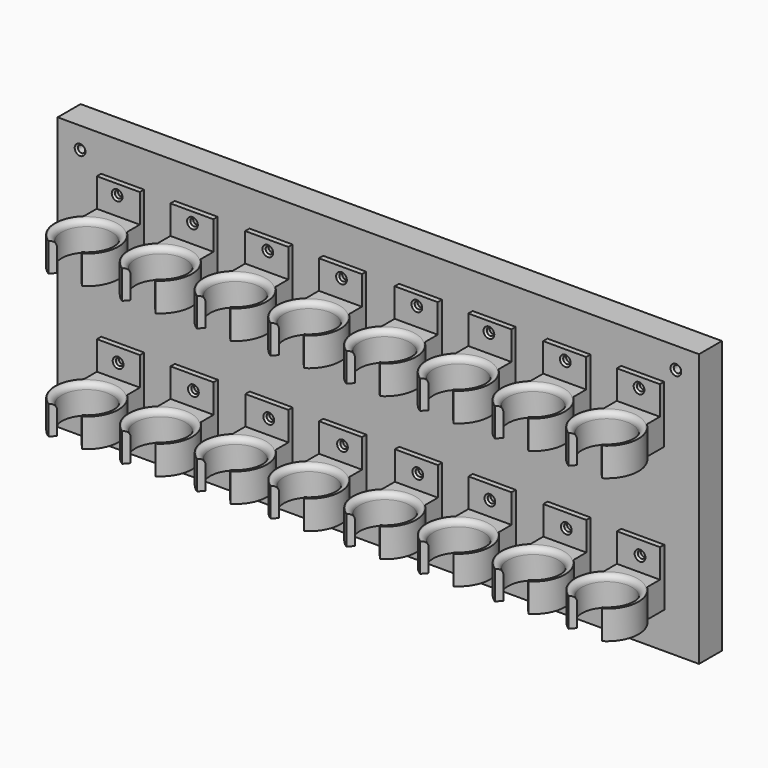
from build123d import *

# Parameters (mm, degrees)
F1_DEPTH          = 25.4
F4_DEPTH          = 25.4
F0_W              = 38.1424913003
F0_H              = 4.7625
F5_DEPTH          = 50.8
F3_W              = 38.1424913003
F3_H              = 4.7625
F6_DEPTH          = 50.8
F9_D              = 6.35
F9_CSINK_D        = 9.525
F9_CSINK_ANGLE    = 90
F9_2_D            = 6.35
F9_2_CSINK_D      = 9.525
F9_2_CSINK_ANGLE  = 90
F9_3_D            = 6.35
F9_3_CSINK_D      = 9.525
F9_3_CSINK_ANGLE  = 90
F9_4_D            = 6.35
F9_4_CSINK_D      = 9.525
F9_4_CSINK_ANGLE  = 90
F9_5_D            = 6.35
F9_5_CSINK_D      = 9.525
F9_5_CSINK_ANGLE  = 90
F9_6_D            = 6.35
F9_6_CSINK_D      = 9.525
F9_6_CSINK_ANGLE  = 90
F9_7_D            = 6.35
F9_7_CSINK_D      = 9.525
F9_7_CSINK_ANGLE  = 90
F9_8_D            = 6.35
F9_8_CSINK_D      = 9.525
F9_8_CSINK_ANGLE  = 90
F12_D             = 6.35
F12_CSINK_D       = 9.525
F12_CSINK_ANGLE   = 90
F12_2_D           = 6.35
F12_2_CSINK_D     = 9.525
F12_2_CSINK_ANGLE = 90
F12_3_D           = 6.35
F12_3_CSINK_D     = 9.525
F12_3_CSINK_ANGLE = 90
F12_4_D           = 6.35
F12_4_CSINK_D     = 9.525
F12_4_CSINK_ANGLE = 90
F12_5_D           = 6.35
F12_5_CSINK_D     = 9.525
F12_5_CSINK_ANGLE = 90
F12_6_D           = 6.35
F12_6_CSINK_D     = 9.525
F12_6_CSINK_ANGLE = 90
F12_7_D           = 6.35
F12_7_CSINK_D     = 9.525
F12_7_CSINK_ANGLE = 90
F12_8_D           = 6.35
F12_8_CSINK_D     = 9.525
F12_8_CSINK_ANGLE = 90
F13_R             = 5.08
F13_2_R           = 5.08
F13_3_R           = 5.08
F13_4_R           = 5.08
F13_5_R           = 5.08
F13_6_R           = 5.08
F13_7_R           = 5.08
F13_8_R           = 5.08
F13_9_R           = 5.08
F13_10_R          = 5.08
F13_11_R          = 5.08
F13_12_R          = 5.08
F13_13_R          = 5.08
F13_14_R          = 5.08
F13_15_R          = 5.08
F13_16_R          = 5.08
F15_W             = 568.5065984726
F15_H             = 241.7119890451
F16_DEPTH         = 25.4
F18_D             = 6.35
F18_CSINK_D       = 9.525
F18_CSINK_ANGLE   = 90


# Not quite as in the source:
# - a feature names something its author has since deleted; it is built from what else it names


with BuildPart() as f1:
    # F0 (on Top) → F1 (new body)
    with BuildSketch(Plane.XY):
        with BuildLine():
            Line((-236.2981056251, -12.180712776), (-274.4405969254, -12.180712776))
            Line((-274.4405969254, -12.180712776), (-274.4405969254, -16.943212776))
            Line((-274.4405969254, -16.943212776), (-274.4405969254, -26.468212776))
            ThreePointArc((-274.4405969254, -26.468212776), (-255.3693512752, -19.0188201484), (-236.2981056251, -26.468212776))
            Line((-236.2981056251, -26.468212776), (-236.2981056251, -16.943212776))
            Line((-236.2981056251, -16.943212776), (-236.2981056251, -12.180712776))
        make_face()
        with BuildLine():
            ThreePointArc((-236.2981056251, -26.468212776), (-255.3693512752, -19.0188201484), (-274.4405969254, -26.468212776))
            ThreePointArc((-274.4405969254, -26.468212776), (-283.3824945845, -49.791985495), (-270.2462375164, -71.0380359006))
            Line((-270.2462375164, -71.0380359006), (-266.2968452207, -66.5087844903))
            ThreePointArc((-266.2968452207, -66.5087844903), (-255.3693512752, -24.9307356072), (-244.4418573298, -66.5087844903))
            Line((-244.4418573298, -66.5087844903), (-240.4924650341, -71.0380359006))
            ThreePointArc((-240.4924650341, -71.0380359006), (-227.356207966, -49.791985495), (-236.2981056251, -26.468212776))
        make_face()
    extrude(amount=F1_DEPTH)

    # F0 (on Top) → F5 (join)
    with BuildSketch(Plane.XY):
        with Locations((-255.3693512752, -9.799462776)):
            Rectangle(F0_W, F0_H)
    extrude(amount=F5_DEPTH)

    # F9 (through all)
    with Locations(Plane.XZ.offset(12.180712776)):
        with Locations((-57.5012685731, 41.7619496584), (-256.4041018486, 41.7619496584), (-122.8343173862, 41.7619496584), (-189.6192133427, 41.7619496584), (206.250667572, 41.7619496584), (73.1648281217, 41.7619496584), (9.2836245894, 41.7619496584), (140.9176290035, 41.7619496584)):
            CounterSinkHole(F9_D / 2, F9_CSINK_D / 2, counter_sink_angle=F9_CSINK_ANGLE)

    # F13
    f13_edges = [f1.edges().sort_by_distance(p)[0] for p in [
        (-255.369351, -24.930736, 25.4),
    ]]
    fillet(f13_edges, radius=F13_R)



with BuildPart() as f1b:
    # F0 (on Top) → F1, piece 2 (new body)
    with BuildSketch(Plane.XY):
        with BuildLine():
            ThreePointArc((-171.0200906615, -26.468212776), (-190.0913363116, -19.0188201484), (-209.1625819618, -26.468212776))
            ThreePointArc((-209.1625819618, -26.468212776), (-218.1044796209, -49.791985495), (-204.9682225528, -71.0380359006))
            Line((-204.9682225528, -71.0380359006), (-201.0188302571, -66.5087844903))
            ThreePointArc((-201.0188302571, -66.5087844903), (-190.0913363116, -24.9307356072), (-179.1638423661, -66.5087844903))
            Line((-179.1638423661, -66.5087844903), (-175.2144500705, -71.0380359006))
            ThreePointArc((-175.2144500705, -71.0380359006), (-162.0781930024, -49.791985495), (-171.0200906615, -26.468212776))
        make_face()
        with BuildLine():
            Line((-171.0200906615, -12.180712776), (-209.1625819618, -12.180712776))
            Line((-209.1625819618, -12.180712776), (-209.1625819618, -16.943212776))
            Line((-209.1625819618, -16.943212776), (-209.1625819618, -26.468212776))
            ThreePointArc((-209.1625819618, -26.468212776), (-190.0913363116, -19.0188201484), (-171.0200906615, -26.468212776))
            Line((-171.0200906615, -26.468212776), (-171.0200906615, -16.943212776))
            Line((-171.0200906615, -16.943212776), (-171.0200906615, -12.180712776))
        make_face()
    extrude(amount=F1_DEPTH)

    # F0 (on Top) → F5, piece 2 (join)
    with BuildSketch(Plane.XY):
        with Locations((-190.0913363116, -9.799462776)):
            Rectangle(F0_W, F0_H)
    extrude(amount=F5_DEPTH)

    # F9#2 (through all)
    with Locations(Plane.XZ.offset(12.180712776)):
        with Locations((-57.5012685731, 41.7619496584), (-256.4041018486, 41.7619496584), (-122.8343173862, 41.7619496584), (-189.6192133427, 41.7619496584), (206.250667572, 41.7619496584), (73.1648281217, 41.7619496584), (9.2836245894, 41.7619496584), (140.9176290035, 41.7619496584)):
            CounterSinkHole(F9_2_D / 2, F9_2_CSINK_D / 2, counter_sink_angle=F9_2_CSINK_ANGLE)

    # F13#2
    f13_2_edges = [f1b.edges().sort_by_distance(p)[0] for p in [
        (-190.091336, -24.930736, 25.4),
    ]]
    fillet(f13_2_edges, radius=F13_2_R)


with BuildPart() as f1c:
    # F0 (on Top) → F1, piece 3 (new body)
    with BuildSketch(Plane.XY):
        with BuildLine():
            Line((-104.6902751007, -12.180712776), (-142.8327664009, -12.180712776))
            Line((-142.8327664009, -12.180712776), (-142.8327664009, -16.943212776))
            Line((-142.8327664009, -16.943212776), (-142.8327664009, -26.468212776))
            ThreePointArc((-142.8327664009, -26.468212776), (-123.7615207508, -19.0188201484), (-104.6902751007, -26.468212776))
            Line((-104.6902751007, -26.468212776), (-104.6902751007, -16.943212776))
            Line((-104.6902751007, -16.943212776), (-104.6902751007, -12.180712776))
        make_face()
        with BuildLine():
            ThreePointArc((-104.6902751007, -26.468212776), (-123.7615207508, -19.0188201484), (-142.8327664009, -26.468212776))
            ThreePointArc((-142.8327664009, -26.468212776), (-151.7746640601, -49.791985495), (-138.638406992, -71.0380359006))
            Line((-138.638406992, -71.0380359006), (-134.6890146963, -66.5087844903))
            ThreePointArc((-134.6890146963, -66.5087844903), (-123.7615207508, -24.9307356072), (-112.8340268053, -66.5087844903))
            Line((-112.8340268053, -66.5087844903), (-108.8846345096, -71.0380359006))
            ThreePointArc((-108.8846345096, -71.0380359006), (-95.7483774415, -49.791985495), (-104.6902751007, -26.468212776))
        make_face()
    extrude(amount=F1_DEPTH)

    # F0 (on Top) → F5, piece 3 (join)
    with BuildSketch(Plane.XY):
        with Locations((-123.7615207508, -9.799462776)):
            Rectangle(F0_W, F0_H)
    extrude(amount=F5_DEPTH)

    # F9#3 (through all)
    with Locations(Plane.XZ.offset(12.180712776)):
        with Locations((-57.5012685731, 41.7619496584), (-256.4041018486, 41.7619496584), (-122.8343173862, 41.7619496584), (-189.6192133427, 41.7619496584), (206.250667572, 41.7619496584), (73.1648281217, 41.7619496584), (9.2836245894, 41.7619496584), (140.9176290035, 41.7619496584)):
            CounterSinkHole(F9_3_D / 2, F9_3_CSINK_D / 2, counter_sink_angle=F9_3_CSINK_ANGLE)

    # F13#3
    f13_3_edges = [f1c.edges().sort_by_distance(p)[0] for p in [
        (-123.761521, -24.930736, 25.4),
    ]]
    fillet(f13_3_edges, radius=F13_3_R)


with BuildPart() as f1d:
    # F0 (on Top) → F1, piece 4 (new body)
    with BuildSketch(Plane.XY):
        with BuildLine():
            ThreePointArc((-39.412260137, -26.468212776), (-58.4835057872, -19.0188201484), (-77.5547514373, -26.468212776))
            ThreePointArc((-77.5547514373, -26.468212776), (-86.4966490964, -49.791985495), (-73.3603920283, -71.0380359006))
            Line((-73.3603920283, -71.0380359006), (-69.4109997327, -66.5087844903))
            ThreePointArc((-69.4109997327, -66.5087844903), (-58.4835057872, -24.9307356072), (-47.5560118417, -66.5087844903))
            Line((-47.5560118417, -66.5087844903), (-43.606619546, -71.0380359006))
            ThreePointArc((-43.606619546, -71.0380359006), (-30.4703624779, -49.791985495), (-39.412260137, -26.468212776))
        make_face()
        with BuildLine():
            Line((-39.412260137, -12.180712776), (-77.5547514373, -12.180712776))
            Line((-77.5547514373, -12.180712776), (-77.5547514373, -16.943212776))
            Line((-77.5547514373, -16.943212776), (-77.5547514373, -26.468212776))
            ThreePointArc((-77.5547514373, -26.468212776), (-58.4835057872, -19.0188201484), (-39.412260137, -26.468212776))
            Line((-39.412260137, -26.468212776), (-39.412260137, -16.943212776))
            Line((-39.412260137, -16.943212776), (-39.412260137, -12.180712776))
        make_face()
    extrude(amount=F1_DEPTH)

    # F0 (on Top) → F5, piece 4 (join)
    with BuildSketch(Plane.XY):
        with Locations((-58.4835057872, -9.799462776)):
            Rectangle(F0_W, F0_H)
    extrude(amount=F5_DEPTH)

    # F9#4 (through all)
    with Locations(Plane.XZ.offset(12.180712776)):
        with Locations((-57.5012685731, 41.7619496584), (-256.4041018486, 41.7619496584), (-122.8343173862, 41.7619496584), (-189.6192133427, 41.7619496584), (206.250667572, 41.7619496584), (73.1648281217, 41.7619496584), (9.2836245894, 41.7619496584), (140.9176290035, 41.7619496584)):
            CounterSinkHole(F9_4_D / 2, F9_4_CSINK_D / 2, counter_sink_angle=F9_4_CSINK_ANGLE)

    # F13#4
    f13_4_edges = [f1d.edges().sort_by_distance(p)[0] for p in [
        (-58.483506, -24.930736, 25.4),
    ]]
    fillet(f13_4_edges, radius=F13_4_R)


with BuildPart() as f1e:
    # F0 (on Top) → F1, piece 5 (new body)
    with BuildSketch(Plane.XY):
        with BuildLine():
            ThreePointArc((27.8059840746, -26.468212776), (8.7347384244, -19.0188201484), (-10.3365072257, -26.468212776))
            ThreePointArc((-10.3365072257, -26.468212776), (-19.2784048848, -49.791985495), (-6.1421478167, -71.0380359006))
            Line((-6.1421478167, -71.0380359006), (-2.192755521, -66.5087844903))
            ThreePointArc((-2.192755521, -66.5087844903), (8.7347384244, -24.9307356072), (19.6622323699, -66.5087844903))
            Line((19.6622323699, -66.5087844903), (23.6116246656, -71.0380359006))
            ThreePointArc((23.6116246656, -71.0380359006), (36.7478817337, -49.791985495), (27.8059840746, -26.468212776))
        make_face()
        with BuildLine():
            Line((27.8059840746, -12.180712776), (-10.3365072257, -12.180712776))
            Line((-10.3365072257, -12.180712776), (-10.3365072257, -16.943212776))
            Line((-10.3365072257, -16.943212776), (-10.3365072257, -26.468212776))
            ThreePointArc((-10.3365072257, -26.468212776), (8.7347384244, -19.0188201484), (27.8059840746, -26.468212776))
            Line((27.8059840746, -26.468212776), (27.8059840746, -16.943212776))
            Line((27.8059840746, -16.943212776), (27.8059840746, -12.180712776))
        make_face()
    extrude(amount=F1_DEPTH)

    # F0 (on Top) → F5, piece 5 (join)
    with BuildSketch(Plane.XY):
        with Locations((8.7347384244, -9.799462776)):
            Rectangle(F0_W, F0_H)
    extrude(amount=F5_DEPTH)

    # F9#5 (through all)
    with Locations(Plane.XZ.offset(12.180712776)):
        with Locations((-57.5012685731, 41.7619496584), (-256.4041018486, 41.7619496584), (-122.8343173862, 41.7619496584), (-189.6192133427, 41.7619496584), (206.250667572, 41.7619496584), (73.1648281217, 41.7619496584), (9.2836245894, 41.7619496584), (140.9176290035, 41.7619496584)):
            CounterSinkHole(F9_5_D / 2, F9_5_CSINK_D / 2, counter_sink_angle=F9_5_CSINK_ANGLE)

    # F13#5
    f13_5_edges = [f1e.edges().sort_by_distance(p)[0] for p in [
        (8.734738, -24.930736, 25.4),
    ]]
    fillet(f13_5_edges, radius=F13_5_R)


with BuildPart() as f1f:
    # F0 (on Top) → F1, piece 6 (new body)
    with BuildSketch(Plane.XY):
        with BuildLine():
            ThreePointArc((93.0839990382, -26.468212776), (74.0127533881, -19.0188201484), (54.9415077379, -26.468212776))
            ThreePointArc((54.9415077379, -26.468212776), (45.9996100788, -49.791985495), (59.1358671469, -71.0380359006))
            Line((59.1358671469, -71.0380359006), (63.0852594426, -66.5087844903))
            ThreePointArc((63.0852594426, -66.5087844903), (74.0127533881, -24.9307356072), (84.9402473335, -66.5087844903))
            Line((84.9402473335, -66.5087844903), (88.8896396292, -71.0380359006))
            ThreePointArc((88.8896396292, -71.0380359006), (102.0258966973, -49.791985495), (93.0839990382, -26.468212776))
        make_face()
        with BuildLine():
            Line((93.0839990382, -12.180712776), (54.9415077379, -12.180712776))
            Line((54.9415077379, -12.180712776), (54.9415077379, -16.943212776))
            Line((54.9415077379, -16.943212776), (54.9415077379, -26.468212776))
            ThreePointArc((54.9415077379, -26.468212776), (74.0127533881, -19.0188201484), (93.0839990382, -26.468212776))
            Line((93.0839990382, -26.468212776), (93.0839990382, -16.943212776))
            Line((93.0839990382, -16.943212776), (93.0839990382, -12.180712776))
        make_face()
    extrude(amount=F1_DEPTH)

    # F0 (on Top) → F5, piece 6 (join)
    with BuildSketch(Plane.XY):
        with Locations((74.0127533881, -9.799462776)):
            Rectangle(F0_W, F0_H)
    extrude(amount=F5_DEPTH)

    # F9#6 (through all)
    with Locations(Plane.XZ.offset(12.180712776)):
        with Locations((-57.5012685731, 41.7619496584), (-256.4041018486, 41.7619496584), (-122.8343173862, 41.7619496584), (-189.6192133427, 41.7619496584), (206.250667572, 41.7619496584), (73.1648281217, 41.7619496584), (9.2836245894, 41.7619496584), (140.9176290035, 41.7619496584)):
            CounterSinkHole(F9_6_D / 2, F9_6_CSINK_D / 2, counter_sink_angle=F9_6_CSINK_ANGLE)

    # F13#6
    f13_6_edges = [f1f.edges().sort_by_distance(p)[0] for p in [
        (74.012753, -24.930736, 25.4),
    ]]
    fillet(f13_6_edges, radius=F13_6_R)


with BuildPart() as f1g:
    # F0 (on Top) → F1, piece 7 (new body)
    with BuildSketch(Plane.XY):
        with BuildLine():
            ThreePointArc((159.413814599, -26.468212776), (140.3425689489, -19.0188201484), (121.2713232988, -26.468212776))
            ThreePointArc((121.2713232988, -26.468212776), (112.3294256396, -49.791985495), (125.4656827077, -71.0380359006))
            Line((125.4656827077, -71.0380359006), (129.4150750034, -66.5087844903))
            ThreePointArc((129.4150750034, -66.5087844903), (140.3425689489, -24.9307356072), (151.2700628944, -66.5087844903))
            Line((151.2700628944, -66.5087844903), (155.2194551901, -71.0380359006))
            ThreePointArc((155.2194551901, -71.0380359006), (168.3557122582, -49.791985495), (159.413814599, -26.468212776))
        make_face()
        with BuildLine():
            Line((159.413814599, -12.180712776), (121.2713232988, -12.180712776))
            Line((121.2713232988, -12.180712776), (121.2713232988, -16.943212776))
            Line((121.2713232988, -16.943212776), (121.2713232988, -26.468212776))
            ThreePointArc((121.2713232988, -26.468212776), (140.3425689489, -19.0188201484), (159.413814599, -26.468212776))
            Line((159.413814599, -26.468212776), (159.413814599, -16.943212776))
            Line((159.413814599, -16.943212776), (159.413814599, -12.180712776))
        make_face()
    extrude(amount=F1_DEPTH)

    # F0 (on Top) → F5, piece 7 (join)
    with BuildSketch(Plane.XY):
        with Locations((140.3425689489, -9.799462776)):
            Rectangle(F0_W, F0_H)
    extrude(amount=F5_DEPTH)

    # F9#7 (through all)
    with Locations(Plane.XZ.offset(12.180712776)):
        with Locations((-57.5012685731, 41.7619496584), (-256.4041018486, 41.7619496584), (-122.8343173862, 41.7619496584), (-189.6192133427, 41.7619496584), (206.250667572, 41.7619496584), (73.1648281217, 41.7619496584), (9.2836245894, 41.7619496584), (140.9176290035, 41.7619496584)):
            CounterSinkHole(F9_7_D / 2, F9_7_CSINK_D / 2, counter_sink_angle=F9_7_CSINK_ANGLE)

    # F13#7
    f13_7_edges = [f1g.edges().sort_by_distance(p)[0] for p in [
        (140.342569, -24.930736, 25.4),
    ]]
    fillet(f13_7_edges, radius=F13_7_R)


with BuildPart() as f1h:
    # F0 (on Top) → F1, piece 8 (new body)
    with BuildSketch(Plane.XY):
        with BuildLine():
            ThreePointArc((224.6918295626, -26.468212776), (205.6205839125, -19.0188201484), (186.5493382624, -26.468212776))
            ThreePointArc((186.5493382624, -26.468212776), (177.6074406032, -49.791985495), (190.7436976713, -71.0380359006))
            Line((190.7436976713, -71.0380359006), (194.693089967, -66.5087844903))
            ThreePointArc((194.693089967, -66.5087844903), (205.6205839125, -24.9307356072), (216.548077858, -66.5087844903))
            Line((216.548077858, -66.5087844903), (220.4974701537, -71.0380359006))
            ThreePointArc((220.4974701537, -71.0380359006), (233.6337272218, -49.791985495), (224.6918295626, -26.468212776))
        make_face()
        with BuildLine():
            Line((224.6918295626, -12.180712776), (186.5493382624, -12.180712776))
            Line((186.5493382624, -12.180712776), (186.5493382624, -16.943212776))
            Line((186.5493382624, -16.943212776), (186.5493382624, -26.468212776))
            ThreePointArc((186.5493382624, -26.468212776), (205.6205839125, -19.0188201484), (224.6918295626, -26.468212776))
            Line((224.6918295626, -26.468212776), (224.6918295626, -16.943212776))
            Line((224.6918295626, -16.943212776), (224.6918295626, -12.180712776))
        make_face()
    extrude(amount=F1_DEPTH)

    # F0 (on Top) → F5, piece 8 (join)
    with BuildSketch(Plane.XY):
        with Locations((205.6205839125, -9.799462776)):
            Rectangle(F0_W, F0_H)
    extrude(amount=F5_DEPTH)

    # F9#8 (through all)
    with Locations(Plane.XZ.offset(12.180712776)):
        with Locations((-57.5012685731, 41.7619496584), (-256.4041018486, 41.7619496584), (-122.8343173862, 41.7619496584), (-189.6192133427, 41.7619496584), (206.250667572, 41.7619496584), (73.1648281217, 41.7619496584), (9.2836245894, 41.7619496584), (140.9176290035, 41.7619496584)):
            CounterSinkHole(F9_8_D / 2, F9_8_CSINK_D / 2, counter_sink_angle=F9_8_CSINK_ANGLE)

    # F13#8
    f13_8_edges = [f1h.edges().sort_by_distance(p)[0] for p in [
        (205.620584, -24.930736, 25.4),
    ]]
    fillet(f13_8_edges, radius=F13_8_R)


with BuildPart() as f4:
    # F3 (on offset) → F4 (new body)
    with BuildSketch(Plane.XY.offset(-127)):
        with BuildLine():
            Line((224.9779318576, -12.3800472473), (186.8354405573, -12.3800472473))
            Line((186.8354405573, -12.3800472473), (186.8354405573, -17.1425472473))
            Line((186.8354405573, -17.1425472473), (186.8354405573, -26.6675472473))
            ThreePointArc((186.8354405573, -26.6675472473), (205.9066862074, -19.2181546196), (224.9779318576, -26.6675472473))
            Line((224.9779318576, -26.6675472473), (224.9779318576, -17.1425472473))
            Line((224.9779318576, -17.1425472473), (224.9779318576, -12.3800472473))
        make_face()
        with BuildLine():
            ThreePointArc((224.9779318576, -26.6675472473), (205.9066862074, -19.2181546196), (186.8354405573, -26.6675472473))
            ThreePointArc((186.8354405573, -26.6675472473), (177.8935428982, -49.9913199663), (191.0297999663, -71.2373703718))
            Line((191.0297999663, -71.2373703718), (194.9791922619, -66.7081189615))
            ThreePointArc((194.9791922619, -66.7081189615), (205.9066862074, -25.1300700784), (216.8341801529, -66.7081189615))
            Line((216.8341801529, -66.7081189615), (220.7835724486, -71.2373703718))
            ThreePointArc((220.7835724486, -71.2373703718), (233.9198295167, -49.9913199663), (224.9779318576, -26.6675472473))
        make_face()
    extrude(amount=F4_DEPTH)

    # F3 (on offset) → F6 (join)
    with BuildSketch(Plane.XY.offset(-127)):
        with Locations((205.9066862074, -9.9987972473)):
            Rectangle(F3_W, F3_H)
    extrude(amount=F6_DEPTH)

    # F12 (through all)
    with Locations(Plane.XZ.offset(12.3800472473)):
        with Locations((-255.3773224354, -88.5276831686), (141.9444084167, -88.5276831686), (-188.5924339294, -88.5276831686), (74.1916075349, -88.5276831686), (207.2774469852, -88.5276831686), (-56.4744891599, -88.5276831686), (-121.8075379729, -88.5276831686), (10.3104040027, -88.5276831686)):
            CounterSinkHole(F12_D / 2, F12_CSINK_D / 2, counter_sink_angle=F12_CSINK_ANGLE)

    # F13#9
    f13_9_edges = [f4.edges().sort_by_distance(p)[0] for p in [
        (205.906686, -25.13007, -101.6),
    ]]
    fillet(f13_9_edges, radius=F13_9_R)


with BuildPart() as f4b:
    # F3 (on offset) → F4, piece 2 (new body)
    with BuildSketch(Plane.XY.offset(-127)):
        with BuildLine():
            ThreePointArc((159.6999168939, -26.6675472473), (140.6286712438, -19.2181546196), (121.5574255937, -26.6675472473))
            ThreePointArc((121.5574255937, -26.6675472473), (112.6155279345, -49.9913199663), (125.7517850026, -71.2373703718))
            Line((125.7517850026, -71.2373703718), (129.7011772983, -66.7081189615))
            ThreePointArc((129.7011772983, -66.7081189615), (140.6286712438, -25.1300700784), (151.5561651893, -66.7081189615))
            Line((151.5561651893, -66.7081189615), (155.505557485, -71.2373703718))
            ThreePointArc((155.505557485, -71.2373703718), (168.6418145531, -49.9913199663), (159.6999168939, -26.6675472473))
        make_face()
        with BuildLine():
            Line((159.6999168939, -12.3800472473), (121.5574255937, -12.3800472473))
            Line((121.5574255937, -12.3800472473), (121.5574255937, -17.1425472473))
            Line((121.5574255937, -17.1425472473), (121.5574255937, -26.6675472473))
            ThreePointArc((121.5574255937, -26.6675472473), (140.6286712438, -19.2181546196), (159.6999168939, -26.6675472473))
            Line((159.6999168939, -26.6675472473), (159.6999168939, -17.1425472473))
            Line((159.6999168939, -17.1425472473), (159.6999168939, -12.3800472473))
        make_face()
    extrude(amount=F4_DEPTH)

    # F3 (on offset) → F6, piece 2 (join)
    with BuildSketch(Plane.XY.offset(-127)):
        with Locations((140.6286712438, -9.9987972473)):
            Rectangle(F3_W, F3_H)
    extrude(amount=F6_DEPTH)

    # F12#2 (through all)
    with Locations(Plane.XZ.offset(12.3800472473)):
        with Locations((-255.3773224354, -88.5276831686), (141.9444084167, -88.5276831686), (-188.5924339294, -88.5276831686), (74.1916075349, -88.5276831686), (207.2774469852, -88.5276831686), (-56.4744891599, -88.5276831686), (-121.8075379729, -88.5276831686), (10.3104040027, -88.5276831686)):
            CounterSinkHole(F12_2_D / 2, F12_2_CSINK_D / 2, counter_sink_angle=F12_2_CSINK_ANGLE)

    # F13#10
    f13_10_edges = [f4b.edges().sort_by_distance(p)[0] for p in [
        (140.628671, -25.13007, -101.6),
    ]]
    fillet(f13_10_edges, radius=F13_10_R)


with BuildPart() as f4c:
    # F3 (on offset) → F4, piece 3 (new body)
    with BuildSketch(Plane.XY.offset(-127)):
        with BuildLine():
            Line((93.3701013331, -12.3800472473), (55.2276100328, -12.3800472473))
            Line((55.2276100328, -12.3800472473), (55.2276100328, -17.1425472473))
            Line((55.2276100328, -17.1425472473), (55.2276100328, -26.6675472473))
            ThreePointArc((55.2276100328, -26.6675472473), (74.298855683, -19.2181546196), (93.3701013331, -26.6675472473))
            Line((93.3701013331, -26.6675472473), (93.3701013331, -17.1425472473))
            Line((93.3701013331, -17.1425472473), (93.3701013331, -12.3800472473))
        make_face()
        with BuildLine():
            ThreePointArc((93.3701013331, -26.6675472473), (74.298855683, -19.2181546196), (55.2276100328, -26.6675472473))
            ThreePointArc((55.2276100328, -26.6675472473), (46.2857123737, -49.9913199663), (59.4219694418, -71.2373703718))
            Line((59.4219694418, -71.2373703718), (63.3713617375, -66.7081189615))
            ThreePointArc((63.3713617375, -66.7081189615), (74.298855683, -25.1300700784), (85.2263496285, -66.7081189615))
            Line((85.2263496285, -66.7081189615), (89.1757419241, -71.2373703718))
            ThreePointArc((89.1757419241, -71.2373703718), (102.3119989923, -49.9913199663), (93.3701013331, -26.6675472473))
        make_face()
    extrude(amount=F4_DEPTH)

    # F3 (on offset) → F6, piece 3 (join)
    with BuildSketch(Plane.XY.offset(-127)):
        with Locations((74.298855683, -9.9987972473)):
            Rectangle(F3_W, F3_H)
    extrude(amount=F6_DEPTH)

    # F12#3 (through all)
    with Locations(Plane.XZ.offset(12.3800472473)):
        with Locations((-255.3773224354, -88.5276831686), (141.9444084167, -88.5276831686), (-188.5924339294, -88.5276831686), (74.1916075349, -88.5276831686), (207.2774469852, -88.5276831686), (-56.4744891599, -88.5276831686), (-121.8075379729, -88.5276831686), (10.3104040027, -88.5276831686)):
            CounterSinkHole(F12_3_D / 2, F12_3_CSINK_D / 2, counter_sink_angle=F12_3_CSINK_ANGLE)

    # F13#11
    f13_11_edges = [f4c.edges().sort_by_distance(p)[0] for p in [
        (74.298856, -25.13007, -101.6),
    ]]
    fillet(f13_11_edges, radius=F13_11_R)


with BuildPart() as f4d:
    # F3 (on offset) → F4, piece 4 (new body)
    with BuildSketch(Plane.XY.offset(-127)):
        with BuildLine():
            Line((28.0920863695, -12.3800472473), (-10.0504049308, -12.3800472473))
            Line((-10.0504049308, -12.3800472473), (-10.0504049308, -17.1425472473))
            Line((-10.0504049308, -17.1425472473), (-10.0504049308, -26.6675472473))
            ThreePointArc((-10.0504049308, -26.6675472473), (9.0208407194, -19.2181546196), (28.0920863695, -26.6675472473))
            Line((28.0920863695, -26.6675472473), (28.0920863695, -17.1425472473))
            Line((28.0920863695, -17.1425472473), (28.0920863695, -12.3800472473))
        make_face()
        with BuildLine():
            ThreePointArc((28.0920863695, -26.6675472473), (9.0208407194, -19.2181546196), (-10.0504049308, -26.6675472473))
            ThreePointArc((-10.0504049308, -26.6675472473), (-18.9923025899, -49.9913199663), (-5.8560455218, -71.2373703718))
            Line((-5.8560455218, -71.2373703718), (-1.9066532261, -66.7081189615))
            ThreePointArc((-1.9066532261, -66.7081189615), (9.0208407194, -25.1300700784), (19.9483346649, -66.7081189615))
            Line((19.9483346649, -66.7081189615), (23.8977269605, -71.2373703718))
            ThreePointArc((23.8977269605, -71.2373703718), (37.0339840286, -49.9913199663), (28.0920863695, -26.6675472473))
        make_face()
    extrude(amount=F4_DEPTH)

    # F3 (on offset) → F6, piece 4 (join)
    with BuildSketch(Plane.XY.offset(-127)):
        with Locations((9.0208407194, -9.9987972473)):
            Rectangle(F3_W, F3_H)
    extrude(amount=F6_DEPTH)

    # F12#4 (through all)
    with Locations(Plane.XZ.offset(12.3800472473)):
        with Locations((-255.3773224354, -88.5276831686), (141.9444084167, -88.5276831686), (-188.5924339294, -88.5276831686), (74.1916075349, -88.5276831686), (207.2774469852, -88.5276831686), (-56.4744891599, -88.5276831686), (-121.8075379729, -88.5276831686), (10.3104040027, -88.5276831686)):
            CounterSinkHole(F12_4_D / 2, F12_4_CSINK_D / 2, counter_sink_angle=F12_4_CSINK_ANGLE)

    # F13#12
    f13_12_edges = [f4d.edges().sort_by_distance(p)[0] for p in [
        (9.020841, -25.13007, -101.6),
    ]]
    fillet(f13_12_edges, radius=F13_12_R)


with BuildPart() as f4e:
    # F3 (on offset) → F4, piece 5 (new body)
    with BuildSketch(Plane.XY.offset(-127)):
        with BuildLine():
            Line((-39.1261578421, -12.3800472473), (-77.2686491424, -12.3800472473))
            Line((-77.2686491424, -12.3800472473), (-77.2686491424, -17.1425472473))
            Line((-77.2686491424, -17.1425472473), (-77.2686491424, -26.6675472473))
            ThreePointArc((-77.2686491424, -26.6675472473), (-58.1974034923, -19.2181546196), (-39.1261578421, -26.6675472473))
            Line((-39.1261578421, -26.6675472473), (-39.1261578421, -17.1425472473))
            Line((-39.1261578421, -17.1425472473), (-39.1261578421, -12.3800472473))
        make_face()
        with BuildLine():
            ThreePointArc((-39.1261578421, -26.6675472473), (-58.1974034923, -19.2181546196), (-77.2686491424, -26.6675472473))
            ThreePointArc((-77.2686491424, -26.6675472473), (-86.2105468015, -49.9913199663), (-73.0742897334, -71.2373703718))
            Line((-73.0742897334, -71.2373703718), (-69.1248974377, -66.7081189615))
            ThreePointArc((-69.1248974377, -66.7081189615), (-58.1974034923, -25.1300700784), (-47.2699095468, -66.7081189615))
            Line((-47.2699095468, -66.7081189615), (-43.3205172511, -71.2373703718))
            ThreePointArc((-43.3205172511, -71.2373703718), (-30.184260183, -49.9913199663), (-39.1261578421, -26.6675472473))
        make_face()
    extrude(amount=F4_DEPTH)

    # F3 (on offset) → F6, piece 5 (join)
    with BuildSketch(Plane.XY.offset(-127)):
        with Locations((-58.1974034923, -9.9987972473)):
            Rectangle(F3_W, F3_H)
    extrude(amount=F6_DEPTH)

    # F12#5 (through all)
    with Locations(Plane.XZ.offset(12.3800472473)):
        with Locations((-255.3773224354, -88.5276831686), (141.9444084167, -88.5276831686), (-188.5924339294, -88.5276831686), (74.1916075349, -88.5276831686), (207.2774469852, -88.5276831686), (-56.4744891599, -88.5276831686), (-121.8075379729, -88.5276831686), (10.3104040027, -88.5276831686)):
            CounterSinkHole(F12_5_D / 2, F12_5_CSINK_D / 2, counter_sink_angle=F12_5_CSINK_ANGLE)

    # F13#13
    f13_13_edges = [f4e.edges().sort_by_distance(p)[0] for p in [
        (-58.197403, -25.13007, -101.6),
    ]]
    fillet(f13_13_edges, radius=F13_13_R)


with BuildPart() as f4f:
    # F3 (on offset) → F4, piece 6 (new body)
    with BuildSketch(Plane.XY.offset(-127)):
        with BuildLine():
            Line((-104.4041728057, -12.3800472473), (-142.546664106, -12.3800472473))
            Line((-142.546664106, -12.3800472473), (-142.546664106, -17.1425472473))
            Line((-142.546664106, -17.1425472473), (-142.546664106, -26.6675472473))
            ThreePointArc((-142.546664106, -26.6675472473), (-123.4754184559, -19.2181546196), (-104.4041728057, -26.6675472473))
            Line((-104.4041728057, -26.6675472473), (-104.4041728057, -17.1425472473))
            Line((-104.4041728057, -17.1425472473), (-104.4041728057, -12.3800472473))
        make_face()
        with BuildLine():
            ThreePointArc((-104.4041728057, -26.6675472473), (-123.4754184559, -19.2181546196), (-142.546664106, -26.6675472473))
            ThreePointArc((-142.546664106, -26.6675472473), (-151.4885617651, -49.9913199663), (-138.352304697, -71.2373703718))
            Line((-138.352304697, -71.2373703718), (-134.4029124014, -66.7081189615))
            ThreePointArc((-134.4029124014, -66.7081189615), (-123.4754184559, -25.1300700784), (-112.5479245104, -66.7081189615))
            Line((-112.5479245104, -66.7081189615), (-108.5985322147, -71.2373703718))
            ThreePointArc((-108.5985322147, -71.2373703718), (-95.4622751466, -49.9913199663), (-104.4041728057, -26.6675472473))
        make_face()
    extrude(amount=F4_DEPTH)

    # F3 (on offset) → F6, piece 6 (join)
    with BuildSketch(Plane.XY.offset(-127)):
        with Locations((-123.4754184559, -9.9987972473)):
            Rectangle(F3_W, F3_H)
    extrude(amount=F6_DEPTH)

    # F12#6 (through all)
    with Locations(Plane.XZ.offset(12.3800472473)):
        with Locations((-255.3773224354, -88.5276831686), (141.9444084167, -88.5276831686), (-188.5924339294, -88.5276831686), (74.1916075349, -88.5276831686), (207.2774469852, -88.5276831686), (-56.4744891599, -88.5276831686), (-121.8075379729, -88.5276831686), (10.3104040027, -88.5276831686)):
            CounterSinkHole(F12_6_D / 2, F12_6_CSINK_D / 2, counter_sink_angle=F12_6_CSINK_ANGLE)

    # F13#14
    f13_14_edges = [f4f.edges().sort_by_distance(p)[0] for p in [
        (-123.475418, -25.13007, -101.6),
    ]]
    fillet(f13_14_edges, radius=F13_14_R)


with BuildPart() as f4g:
    # F3 (on offset) → F4, piece 7 (new body)
    with BuildSketch(Plane.XY.offset(-127)):
        with BuildLine():
            Line((-170.7339883666, -12.3800472473), (-208.8764796668, -12.3800472473))
            Line((-208.8764796668, -12.3800472473), (-208.8764796668, -17.1425472473))
            Line((-208.8764796668, -17.1425472473), (-208.8764796668, -26.6675472473))
            ThreePointArc((-208.8764796668, -26.6675472473), (-189.8052340167, -19.2181546196), (-170.7339883666, -26.6675472473))
            Line((-170.7339883666, -26.6675472473), (-170.7339883666, -17.1425472473))
            Line((-170.7339883666, -17.1425472473), (-170.7339883666, -12.3800472473))
        make_face()
        with BuildLine():
            ThreePointArc((-170.7339883666, -26.6675472473), (-189.8052340167, -19.2181546196), (-208.8764796668, -26.6675472473))
            ThreePointArc((-208.8764796668, -26.6675472473), (-217.818377326, -49.9913199663), (-204.6821202579, -71.2373703718))
            Line((-204.6821202579, -71.2373703718), (-200.7327279622, -66.7081189615))
            ThreePointArc((-200.7327279622, -66.7081189615), (-189.8052340167, -25.1300700784), (-178.8777400712, -66.7081189615))
            Line((-178.8777400712, -66.7081189615), (-174.9283477755, -71.2373703718))
            ThreePointArc((-174.9283477755, -71.2373703718), (-161.7920907074, -49.9913199663), (-170.7339883666, -26.6675472473))
        make_face()
    extrude(amount=F4_DEPTH)

    # F3 (on offset) → F6, piece 7 (join)
    with BuildSketch(Plane.XY.offset(-127)):
        with Locations((-189.8052340167, -9.9987972473)):
            Rectangle(F3_W, F3_H)
    extrude(amount=F6_DEPTH)

    # F12#7 (through all)
    with Locations(Plane.XZ.offset(12.3800472473)):
        with Locations((-255.3773224354, -88.5276831686), (141.9444084167, -88.5276831686), (-188.5924339294, -88.5276831686), (74.1916075349, -88.5276831686), (207.2774469852, -88.5276831686), (-56.4744891599, -88.5276831686), (-121.8075379729, -88.5276831686), (10.3104040027, -88.5276831686)):
            CounterSinkHole(F12_7_D / 2, F12_7_CSINK_D / 2, counter_sink_angle=F12_7_CSINK_ANGLE)

    # F13#15
    f13_15_edges = [f4g.edges().sort_by_distance(p)[0] for p in [
        (-189.805234, -25.13007, -101.6),
    ]]
    fillet(f13_15_edges, radius=F13_15_R)


with BuildPart() as f4h:
    # F3 (on offset) → F4, piece 8 (new body)
    with BuildSketch(Plane.XY.offset(-127)):
        with BuildLine():
            Line((-236.0120033302, -12.3800472473), (-274.1544946305, -12.3800472473))
            Line((-274.1544946305, -12.3800472473), (-274.1544946305, -17.1425472473))
            Line((-274.1544946305, -17.1425472473), (-274.1544946305, -26.6675472473))
            ThreePointArc((-274.1544946305, -26.6675472473), (-255.0832489803, -19.2181546196), (-236.0120033302, -26.6675472473))
            Line((-236.0120033302, -26.6675472473), (-236.0120033302, -17.1425472473))
            Line((-236.0120033302, -17.1425472473), (-236.0120033302, -12.3800472473))
        make_face()
        with BuildLine():
            ThreePointArc((-236.0120033302, -26.6675472473), (-255.0832489803, -19.2181546196), (-274.1544946305, -26.6675472473))
            ThreePointArc((-274.1544946305, -26.6675472473), (-283.0963922896, -49.9913199663), (-269.9601352215, -71.2373703718))
            Line((-269.9601352215, -71.2373703718), (-266.0107429258, -66.7081189615))
            ThreePointArc((-266.0107429258, -66.7081189615), (-255.0832489803, -25.1300700784), (-244.1557550348, -66.7081189615))
            Line((-244.1557550348, -66.7081189615), (-240.2063627392, -71.2373703718))
            ThreePointArc((-240.2063627392, -71.2373703718), (-227.070105671, -49.9913199663), (-236.0120033302, -26.6675472473))
        make_face()
    extrude(amount=F4_DEPTH)

    # F3 (on offset) → F6, piece 8 (join)
    with BuildSketch(Plane.XY.offset(-127)):
        with Locations((-255.0832489803, -9.9987972473)):
            Rectangle(F3_W, F3_H)
    extrude(amount=F6_DEPTH)

    # F12#8 (through all)
    with Locations(Plane.XZ.offset(12.3800472473)):
        with Locations((-255.3773224354, -88.5276831686), (141.9444084167, -88.5276831686), (-188.5924339294, -88.5276831686), (74.1916075349, -88.5276831686), (207.2774469852, -88.5276831686), (-56.4744891599, -88.5276831686), (-121.8075379729, -88.5276831686), (10.3104040027, -88.5276831686)):
            CounterSinkHole(F12_8_D / 2, F12_8_CSINK_D / 2, counter_sink_angle=F12_8_CSINK_ANGLE)

    # F13#16
    f13_16_edges = [f4h.edges().sort_by_distance(p)[0] for p in [
        (-255.083249, -25.13007, -101.6),
    ]]
    fillet(f13_16_edges, radius=F13_16_R)


with BuildPart() as f1_1:
    add(f1.part)

    add(f1b.part)  # F16 merges F1b

    add(f1c.part)  # F16 merges F1c

    add(f1d.part)  # F16 merges F1d

    add(f1e.part)  # F16 merges F1e

    add(f1f.part)  # F16 merges F1f

    add(f1g.part)  # F16 merges F1g

    add(f1h.part)  # F16 merges F1h
    # F15 (on offset) → F16 (join)
    with BuildSketch(Plane(origin=(0, -7.418212776, 0), x_dir=(-1, 0, 0), z_dir=(0, 1, 0))):
        with Locations((28.6536216736, -38.5328605771)):
            Rectangle(F15_W, F15_H)
    extrude(amount=F16_DEPTH)

    # F18 (through all)
    with Locations(Plane.XZ.offset(7.418212776)):
        with Locations((-293.0452525616, 63.374646008), (235.1121604443, 63.374646008)):
            CounterSinkHole(F18_D / 2, F18_CSINK_D / 2, counter_sink_angle=F18_CSINK_ANGLE)


solid = Compound([f4.part, f4b.part, f4c.part, f4d.part, f4e.part, f4f.part, f4g.part, f4h.part, f1_1.part])
